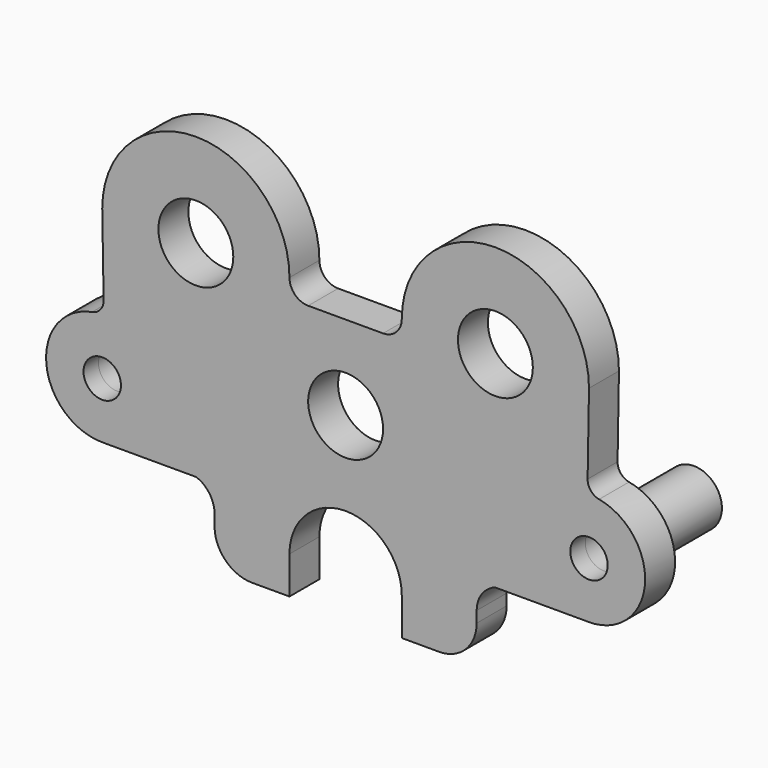
from build123d import *

# Parameters (mm, degrees)
F0_R     = 9.525
F0_R_2   = 12.7
F0_R_3   = 6.35
F1_DEPTH = 6.35
F2_R     = 12.7
F3_R     = 4.7625
F4_R     = 6.34999
F5_DEPTH = 38.1


# Not quite as in the source:
# - a fillet or chamfer is up to 0.001 mm smaller than in the source, because OpenCascade refuses the exact size


with BuildPart() as f1:
    # F0 (on Front) → F1 (new body, symmetric)
    with BuildSketch(Plane.XZ):
        with BuildLine():
            Line((-19.05, -60.325), (-19.05, -47.625))
            ThreePointArc((-19.05, -47.625), (0, -28.575), (19.05, -47.625))
            Line((19.05, -47.625), (19.05, -60.325))
            Line((19.05, -60.325), (44.45, -60.325))
            Line((44.45, -60.325), (44.45, -43.8458790377))
            ThreePointArc((44.45, -43.8458790377), (46.1544838519, -38.4084943559), (50.6579059691, -34.9171326425))
            Line((50.6579059691, -34.9171326425), (82.0025655956, -34.9171326425))
            ThreePointArc((82.0025655956, -34.9171326425), (101.6, -15.875), (82.0025655956, 3.1671326425))
            Line((82.0025655956, 3.1671326425), (82.55, 34.925))
            ThreePointArc((82.55, 34.925), (50.8, 66.675), (19.05, 34.925))
            Line((19.05, 34.925), (19.05, 28.575))
            Line((19.05, 28.575), (-19.05, 28.575))
            Line((-19.05, 28.575), (-19.05, 34.925))
            ThreePointArc((-19.05, 34.925), (-50.8, 66.675), (-82.55, 34.925))
            Line((-82.55, 34.925), (-82.0025655956, 3.1671326425))
            ThreePointArc((-82.0025655956, 3.1671326425), (-101.6, -15.875), (-82.0025655956, -34.9171326425))
            Line((-82.0025655956, -34.9171326425), (-50.6579059691, -34.9171326425))
            ThreePointArc((-50.6579059691, -34.9171326425), (-46.1544838519, -38.4084943559), (-44.45, -43.8458790377))
            Line((-44.45, -43.8458790377), (-44.45, -60.325))
            Line((-44.45, -60.325), (-19.05, -60.325))
        make_face()
        with Locations((-82.55, -15.875)):
            Circle(F0_R, mode=Mode.SUBTRACT)
        Circle(F0_R_2, mode=Mode.SUBTRACT)
        with Locations((82.55, -15.875)):
            Circle(F0_R, mode=Mode.SUBTRACT)
        with Locations((-50.8, 34.925)):
            Circle(F0_R_2, mode=Mode.SUBTRACT)
        with Locations((50.8, 34.925)):
            Circle(F0_R_2, mode=Mode.SUBTRACT)
        with Locations((-82.55, -15.875)):
            Circle(F0_R)
        with Locations((-82.55, -15.875)):
            Circle(F0_R_3, mode=Mode.SUBTRACT)
        with Locations((82.55, -15.875)):
            Circle(F0_R)
        with Locations((82.55, -15.875)):
            Circle(F0_R_3, mode=Mode.SUBTRACT)
    extrude(amount=F1_DEPTH, both=True)

    # F2
    f2_edges = [f1.edges().sort_by_distance(p)[0] for p in [
        (-44.45, 0, -60.325),
        (44.45, 0, -60.325),
    ]]
    fillet(f2_edges, radius=F2_R)

    # F3
    f3_edges = [f1.edges().sort_by_distance(p)[0] for p in [
        (-82.002566, 0, 3.167133),
        (82.002566, 0, 3.167133),
    ]]
    fillet(f3_edges, radius=F3_R)

    # F4 (radius 6.35 in the source; OpenCascade refuses exactly that, so slightly less here)
    f4_edges = [f1.edges().sort_by_distance(p)[0] for p in [
        (-19.05, 0, 28.575),
        (19.05, 0, 28.575),
    ]]
    fillet(f4_edges, radius=F4_R)

    # F0 (on Front) → F5 (join)
    with BuildSketch(Plane.XZ):
        with Locations((-82.55, -15.875)):
            Circle(F0_R)
        with Locations((-82.55, -15.875)):
            Circle(F0_R_3, mode=Mode.SUBTRACT)
        with Locations((82.55, -15.875)):
            Circle(F0_R)
        with Locations((82.55, -15.875)):
            Circle(F0_R_3, mode=Mode.SUBTRACT)
    extrude(amount=-F5_DEPTH)


solid = f1.part
